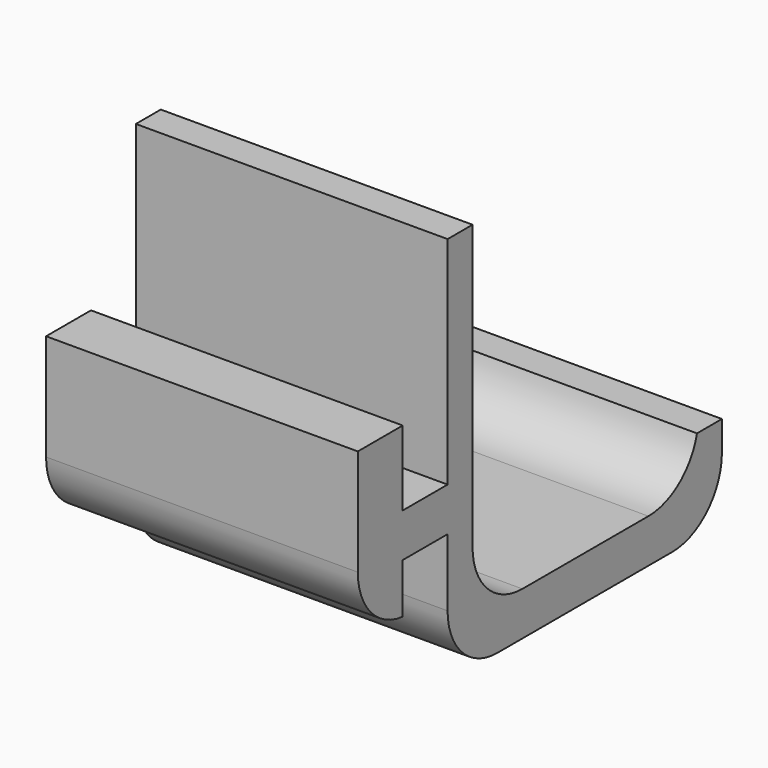
from build123d import *

# Parameters (mm, degrees)
F0_W        = 2.5
F0_H        = 3.8657399043
F1_DEPTH    = 25
F2_T1_DEPTH = 25
F2_T3_DEPTH = 25
F2_T5_DEPTH = 50
F2_T7_DEPTH = 50
F3_T1_DEPTH = 49.8746859277


# Not quite as in the source:
# - a fillet or chamfer that OpenCascade refuses, or shapes differently, is made with other operations: its cross-section is extruded or revolved along the edge and cut away or added


with BuildPart() as f1:
    # F0 (on Right) → F1 (new body)
    with BuildSketch(Plane.YZ):
        Polygon((4.5518016368, 4.6355622155), (0.0518016368, 4.6355622155), (0.0518016368, -8.8644377845), (4.5518016368, -8.8644377845), (4.5518016368, -4.8644377845), (9.0518016368, -4.8644377845), (9.0518016368, -15.2773326263), (11.5518016368, -15.2773326263), (11.5518016368, -11.7773326263), (11.5518016368, 15.966644237), (9.0518016368, 15.966644237), (9.0518016368, -1.3644377845), (4.5518016368, -1.3644377845), align=None)
        Polygon((11.5518016368, -11.7773326263), (11.5518016368, -15.2773326263), (36.5518016368, -15.2773326263), (36.5518016368, -11.7773326263), (34.0518016368, -11.7773326263), align=None)
        with Locations((35.3018016368, -9.8444626741)):
            Rectangle(F0_W, F0_H)
    extrude(amount=F1_DEPTH)

    # F2: fillet of radius 5 on 4 edges, made by hand

    # F2_s2 → F2_t1 (join)
    with BuildSketch(Plane.YZ):
        with BuildLine():
            ThreePointArc((34.0518016368, -7.9115927219), (32.2909091759, -10.6934084988), (29.1821554448, -11.7773326263))
            Line((29.1821554448, -11.7773326263), (34.0518016368, -11.7773326263))
            Line((34.0518016368, -11.7773326263), (34.0518016368, -7.9115927219))
        make_face()
    extrude(amount=F2_T1_DEPTH)

    # F2_s4 → F2_t3 (join)
    with BuildSketch(Plane.YZ):
        with BuildLine():
            ThreePointArc((16.5518016368, -11.7773326263), (13.0162677309, -10.3128665322), (11.5518016368, -6.7773326263))
            Line((11.5518016368, -6.7773326263), (11.5518016368, -11.7773326263))
            Line((11.5518016368, -11.7773326263), (16.5518016368, -11.7773326263))
        make_face()
    extrude(amount=F2_T3_DEPTH)

    # F2_s6 → F2_t5 (cut)
    with BuildSketch(Plane.YZ.offset(-12.5)):
        with BuildLine():
            ThreePointArc((9.0518016368, -10.2773326263), (10.5162677309, -13.8128665322), (14.0518016368, -15.2773326263))
            Line((14.0518016368, -15.2773326263), (9.0518016368, -15.2773326263))
            Line((9.0518016368, -15.2773326263), (9.0518016368, -10.2773326263))
        make_face()
    extrude(amount=F2_T5_DEPTH, mode=Mode.SUBTRACT)

    # F2_s8 → F2_t7 (cut)
    with BuildSketch(Plane.YZ.offset(-12.5)):
        with BuildLine():
            ThreePointArc((36.5518016368, -10.2773326263), (35.0873355427, -13.8128665322), (31.5518016368, -15.2773326263))
            Line((31.5518016368, -15.2773326263), (36.5518016368, -15.2773326263))
            Line((36.5518016368, -15.2773326263), (36.5518016368, -10.2773326263))
        make_face()
    extrude(amount=F2_T7_DEPTH, mode=Mode.SUBTRACT)

    # F3: fillet of radius 5 on 1 edges, made by hand

    # F3_s2 → F3_t1 (cut)
    with BuildSketch(Plane.YZ.offset(-12.4373429638)):
        with BuildLine():
            ThreePointArc((0.0518016368, -3.889500599), (1.3437023933, -7.2436025653), (4.5518016368, -8.8644377845))
            Line((4.5518016368, -8.8644377845), (0.0518016368, -8.8644377845))
            Line((0.0518016368, -8.8644377845), (0.0518016368, -3.889500599))
        make_face()
    extrude(amount=F3_T1_DEPTH, mode=Mode.SUBTRACT)


solid = f1.part
